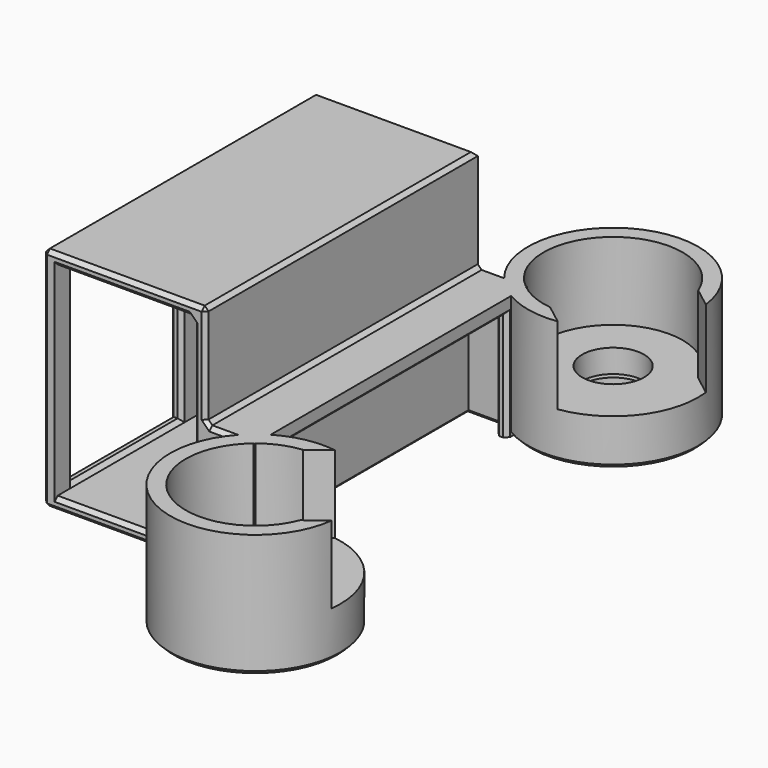
from build123d import *

# Parameters (mm, degrees)
F0_W      = 21
F0_H      = 29.3000006603
F0_W_2    = 18
F0_H_2    = 26.3
F1_DEPTH  = 44
F3_W      = 1.5
F3_H      = 37.5
F4_DEPTH  = 2
F5_DEPTH  = 16
F10_R     = 1
F12_DEPTH = 10
F16_W     = 17.5
F16_H     = 25.3000006603
F17_DEPTH = 1.5
F18_SIZE  = 0.49999


# Not quite as in the source:
# - a fillet or chamfer is up to 0.001 mm smaller than in the source, because OpenCascade refuses the exact size


with BuildPart() as f1:
    # F0 (on Front) → F1 (new body)
    with BuildSketch(Plane.XZ):
        with Locations((-9, -3.302e-07)):
            Rectangle(F0_W, F0_H)
        with Locations((-9, 0)):
            Rectangle(F0_W_2, F0_H_2, mode=Mode.SUBTRACT)
    extrude(amount=F1_DEPTH)

    # F3 (on offset) → F4 (join)
    with BuildSketch(Plane(origin=(0, 0, 1.3499993397), x_dir=(1, 0, 0), z_dir=(0, 0, -1))):
        Polygon((1.5, 1.5), (1.5, 0), (7.8722483143, 0), (7.8722483143, 3.25), (6.3722483143, 3.25), (6.3722483143, 1.5), align=None)
        with Locations((7.1222483143, 22)):
            Rectangle(F3_W, F3_H)
        Polygon((1.5, 42.5), (1.5, 1.5), (6.3722483143, 1.5), (6.3722483143, 3.25), (6.3722483143, 40.75), (6.3722483143, 42.5), align=None)
        Polygon((1.5, 44), (1.5, 42.5), (6.3722483143, 42.5), (6.3722483143, 40.75), (7.8722483143, 40.75), (7.8722483143, 44), align=None)
    extrude(amount=F4_DEPTH)

    # F3 (on offset) → F5 (join, through all)
    with BuildSketch(Plane(origin=(0, 0, 1.3499993397), x_dir=(1, 0, 0), z_dir=(0, 0, -1))):
        Polygon((1.5, 1.5), (1.5, 0), (7.8722483143, 0), (7.8722483143, 3.25), (6.3722483143, 3.25), (6.3722483143, 1.5), align=None)
        Polygon((1.5, 44), (1.5, 42.5), (6.3722483143, 42.5), (6.3722483143, 40.75), (7.8722483143, 40.75), (7.8722483143, 44), align=None)
    extrude(amount=F5_DEPTH)

    # F8 (on offset) → F9 (revolve)
    with BuildSketch(Plane.YZ.offset(13.4722483143)):
        Polygon((10.9, -8.6500006603), (10.9, -11.6500006603), (15.4, -11.6500006603), (15.4, -14.1500006603), (15.9, -14.6500006603), (17.4, -14.6500006603), (17.9, -14.1500006603), (17.9, 1.3499993397), (15.9, 1.3499993397), (15.9, -8.6500006603), align=None)
    revolve(axis=Axis((13.4722483143, 6.9, -10.1500006603), (0, 0, -1)))

    # F10
    f10_edges = [f1.edges().sort_by_distance(p)[0] for p in [
        (13.472248, -1.6, -11.650001),
    ]]
    fillet(f10_edges, radius=F10_R)

    # F11 (on face) → F12 (cut)
    with BuildSketch(Plane.XY.offset(1.3499993397)):
        with BuildLine():
            Line((24.3916150789, 8.2294470504), (21.8554232448, 10.1745042503))
            ThreePointArc((21.8554232448, 10.1745042503), (20.6138305896, 1.4229750224), (12.4836249498, -2.0455365319))
            Line((12.4836249498, -2.0455365319), (15.019816784, -3.9905937318))
            ThreePointArc((15.019816784, -3.9905937318), (22.200848873, 0.2058583608), (24.3916150789, 8.2294470504))
        make_face()
    extrude(amount=-F12_DEPTH, mode=Mode.SUBTRACT)


with BuildPart() as f9:
    # F8 (on offset) → F9, piece 2 (revolve)
    with BuildSketch(Plane.YZ.offset(13.4722483143)):
        Polygon((10.9, -12.0500006603), (10.9, -14.6500006603), (11.5, -14.6500006603), (11.5, -12.6500006603), (13.8, -12.6500006603), (13.8, -14.6500006603), (14.4, -14.6500006603), (14.4, -12.0500006603), (11.5, -12.0500006603), align=None)
    revolve(axis=Axis((13.4722483143, 6.9, -10.1500006603), (0, 0, -1)))


with BuildPart() as f14_1:
    # F14: instance of F1
    add(f1.part.mirror(Plane(origin=(0, -22, 0), x_dir=(-1, 0, 0), z_dir=(0, 1, 0))))

    # F15: union F1
    add(f1.part)

    # F16 (on face) → F17 (cut, through all)
    with BuildSketch(Plane(origin=(-19.5, 0, 0), x_dir=(0, -1, 0), z_dir=(-1, 0, 0))):
        with Locations((11.75, -3.302e-07)):
            Rectangle(F16_W, F16_H)
        with Locations((32.25, -3.302e-07)):
            Rectangle(F16_W, F16_H)
    extrude(amount=-F17_DEPTH, mode=Mode.SUBTRACT)

    # F18 (size 0.5 in the source; OpenCascade refuses exactly that, so slightly less here)
    f18_edges = [f14_1.edges().sort_by_distance(p)[0] for p in [
        (-19.5, -22, 14.65),
        (-19.5, -22, -14.650001),
        (-19.5, 0, 0),
        (-19.5, -44, 0),
        (1.5, -22, 14.65),
        (-9, 0, 14.65),
        (-9, -44, 14.65),
        (-19.5, -23.5, 0),
        (-19.5, -32.25, 12.65),
        (-18, -32.25, 12.65),
        (-18, -23.5, 0),
        (-18, -20.5, 0),
        (-18, -3, 0),
        (-18, 0, 0),
        (-18, -32.25, -12.650001),
        (-18, -11.75, -12.650001),
        (-18, -41, 0),
        (-9, -44, -13.15),
        (-9, 0, -13.15),
        (0, 0, 0),
        (0, -44, 0),
        (0, -22, -13.15),
        (0, -22, 13.15),
        (1.5, -22, 1.349999),
        (1.5, -44, 8),
        (7.872248, -3.25, -7.650001),
        (7.872248, -22, -0.650001),
        (7.872248, -40.75, -7.650001),
        (6.372248, -40.75, -7.650001),
        (6.372248, -41.625, -14.650001),
        (-6.971148, -44, -14.650001),
        (1.5, -22, -14.650001),
        (3.936124, -1.5, -14.650001),
        (6.372248, -3.25, -7.650001),
        (-19.5, -11.75, 12.65),
        (-18, -11.75, 12.65),
        (-19.5, -20.5, 0),
        (-19.5, -41, 0),
        (-19.5, -3, 0),
        (-19.5, -11.75, -12.650001),
        (-19.5, -32.25, -12.650001),
        (-6.971148, 0, -14.650001),
        (3.202726, -44, 1.349999),
        (-9, -44, 13.15),
        (-9, 0, 13.15),
    ]]
    chamfer(f18_edges, length=F18_SIZE)


with BuildPart() as f14_2:
    # F14: instance of F9
    add(f9.part.mirror(Plane(origin=(0, -22, 0), x_dir=(-1, 0, 0), z_dir=(0, 1, 0))))


solid = Compound([f9.part, f14_1.part, f14_2.part])
